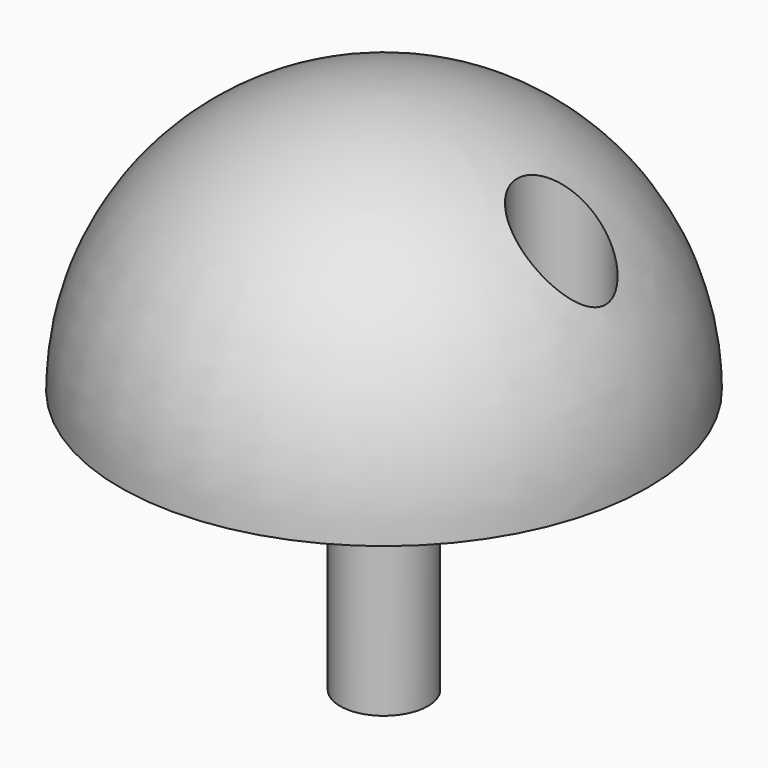
from build123d import *

# Parameters (mm, degrees)
F2_R     = 6.35
F3_DEPTH = 50.8


# Not quite as in the source:
# - ends of sketch curves that miss each other by under 0.0002 mm in the source are joined


with BuildPart() as f1:
    # F0 (on Front) → F1 (revolve)
    with BuildSketch(Plane.XZ):
        with BuildLine():
            Line((0, 76.2), (0, 0))
            Line((0, 0), (6.3499988439, 0))
            Line((6.3499988439, 0), (6.3499988439, 38.1))
            Line((6.3499988439, 38.1), (38.0999988439, 38.1))
            ThreePointArc((38.0999988439, 38.1), (26.9407683632, 65.0407683632), (0, 76.2))
        make_face()
    revolve(axis=Axis((0, 0, 38.1), (0, 0, 1)))

    # F2 (on face) → F3 (cut)
    with BuildSketch(Plane(origin=(0, 0, 38.1), x_dir=(1, 0, 0), z_dir=(0, 0, -1))):
        with Locations((25.3987728004, -0.2495626229)):
            Circle(F2_R)
    extrude(amount=-F3_DEPTH, mode=Mode.SUBTRACT)


solid = f1.part
